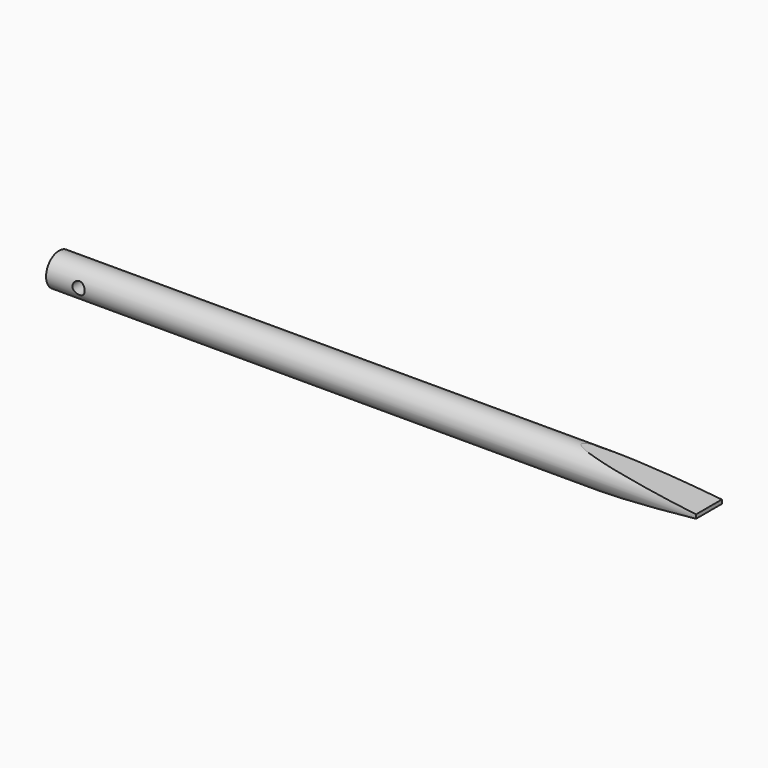
from build123d import *

# Parameters (mm, degrees)
F0_R          = 3.175
F1_DEPTH      = 127
F3_DEPTH      = 25.4
F3_DEPTH_BACK = 25.4
F4_R          = 1.1938
F6_DEPTH      = 3.175
F6_DEPTH_BACK = 3.175


# Not quite as in the source:
# - the program builds the solid bodies; features that only make, move or delete a surface that nothing else refers to are left out


with BuildPart() as f1:
    # F0 (on Right) → F1 (new body)
    with BuildSketch(Plane.YZ):
        Circle(F0_R)
    extrude(amount=-F1_DEPTH)

    # F2 (on Front) → F3 (cut, two sides)
    with BuildSketch(Plane.XZ) as f3_sk:
        Polygon((-25.4, 3.2325035427), (0, 0.381), (0, 3.2325035427), align=None)
        Polygon((0, -3.2135259826), (0, -0.381), (-25.4, -3.2325035427), align=None)
    extrude(amount=-F3_DEPTH, mode=Mode.SUBTRACT)
    extrude(f3_sk.sketch, amount=F3_DEPTH_BACK, mode=Mode.SUBTRACT)

    # F4 (on Front) → F6 (cut, two sides)
    with BuildSketch(Plane.XZ) as f6_sk:
        with Locations((-120.65, 0)):
            Circle(F4_R)
    extrude(amount=F6_DEPTH, mode=Mode.SUBTRACT)
    extrude(f6_sk.sketch, amount=-F6_DEPTH_BACK, mode=Mode.SUBTRACT)


solid = f1.part
